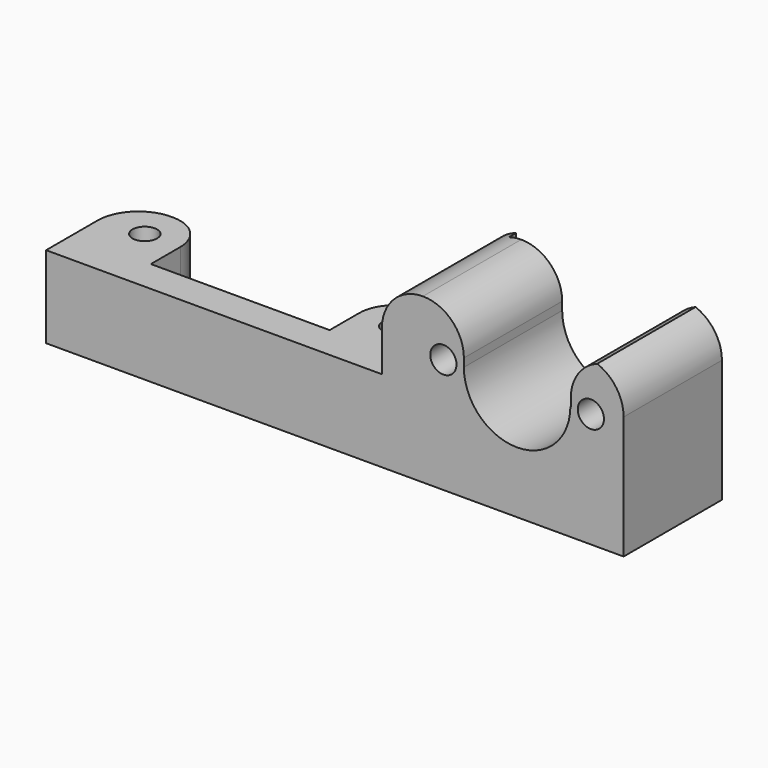
from build123d import *

# Parameters (mm, degrees)
F0_R        = 1.5
F1_DEPTH    = 10
F2_DEPTH    = 20
F4_R        = 1.6
F5_DEPTH    = 15
F6_T1_DEPTH = 40
F6_T3_DEPTH = 41.1
F6_T5_DEPTH = 35.7954738485


# Not quite as in the source:
# - a fillet or chamfer that OpenCascade refuses, or shapes differently, is made with other operations: its cross-section is extruded or revolved along the edge and cut away or added


with BuildPart() as f1:
    # F0 (on Top) → F1 (new body)
    with BuildSketch(Plane.XY):
        with BuildLine():
            Line((-15.25, 4.3355262056), (-20.5, 4.5))
            Line((-20.5, 4.5), (-20.5, -4.5))
            Line((-20.5, -4.5), (-10.9144737944, -4.5))
            Line((-10.9144737944, -4.5), (-10.9144737944, 0))
            ThreePointArc((-10.9144737944, 0), (-12.18432002, 3.06567998), (-15.25, 4.3355262056))
        make_face()
        with Locations((-15.25, 0)):
            Circle(F0_R, mode=Mode.SUBTRACT)
        Polygon((20.5, -8.5), (20.5, -4.5), (10.9144737944, -4.5), (-10.9144737944, -4.5), (-20.5, -4.5), (-20.5, -8.5), align=None)
        with BuildLine():
            Line((20.5, -4.5), (20.5, 4.5))
            Line((20.5, 4.5), (15.25, 4.3355262056))
            ThreePointArc((15.25, 4.3355262056), (12.18432002, 3.06567998), (10.9144737944, 0))
            Line((10.9144737944, 0), (10.9144737944, -4.5))
            Line((10.9144737944, -4.5), (20.5, -4.5))
        make_face()
        with Locations((15.25, 0)):
            Circle(F0_R, mode=Mode.SUBTRACT)
    extrude(amount=F1_DEPTH)


with BuildPart() as f2:
    # F0 (on Top) → F2 (new body)
    with BuildSketch(Plane.XY):
        Polygon((20.5, 7.6), (20.5, 4.5), (20.5, -4.5), (20.5, -8.5), (24, -8.5), (24, 0), (24, 7.6), align=None)
    extrude(amount=F2_DEPTH)


with BuildPart() as f1_1:
    add(f1.part)

    # F3: union F2
    add(f2.part)

    # F4 (on face) → F5 (join)
    with BuildSketch(Plane.XZ.offset(8.5)):
        with BuildLine():
            Line((24, 14), (24, 0))
            Line((24, 0), (50, 0))
            Line((50, 0), (50, 14))
            Line((50, 14), (50, 20))
            Line((50, 20), (43.5623936355, 20))
            Line((43.5623936355, 20), (43.5623936355, 14))
            Line((43.5623936355, 14), (43.5, 14))
            ThreePointArc((43.5, 14), (37, 7.5), (30.5, 14))
            Line((30.5, 14), (30.5, 20))
            Line((30.5, 20), (24, 20))
            Line((24, 20), (24, 14))
        make_face()
        with Locations((28, 14)):
            Circle(F4_R, mode=Mode.SUBTRACT)
        with Locations((46, 14)):
            Circle(F4_R, mode=Mode.SUBTRACT)
    extrude(amount=-F5_DEPTH)

    # F6: fillet of radius 5 on 5 edges, made by hand

    # F6_s2 → F6_t1 (cut)
    with BuildSketch(Plane.XZ.offset(-19)):
        with BuildLine():
            ThreePointArc((43.5623936355, 15), (45.0268597296, 18.5355339059), (48.5623936355, 20))
            Line((48.5623936355, 20), (43.5623936355, 20))
            Line((43.5623936355, 20), (43.5623936355, 15))
        make_face()
        with BuildLine():
            ThreePointArc((45, 20), (48.5355339059, 18.5355339059), (50, 15))
            Line((50, 15), (50, 20))
            Line((50, 20), (45, 20))
        make_face()
        with BuildLine():
            ThreePointArc((30.5, 15), (29.0355339059, 18.5355339059), (25.5, 20))
            Line((25.5, 20), (30.5, 20))
            Line((30.5, 20), (30.5, 15))
        make_face()
    extrude(amount=F6_T1_DEPTH, mode=Mode.SUBTRACT)

    # F6_s4 → F6_t3 (cut)
    with BuildSketch(Plane.XZ.offset(-20.1)):
        with BuildLine():
            ThreePointArc((20.5, 15), (21.9644660941, 18.5355339059), (25.5, 20))
            Line((25.5, 20), (20.5, 20))
            Line((20.5, 20), (20.5, 15))
        make_face()
    extrude(amount=F6_T3_DEPTH, mode=Mode.SUBTRACT)

    # F6_s6 → F6_t5 (cut)
    with BuildSketch(Plane.XY.offset(-12.8977369243)):
        with BuildLine():
            ThreePointArc((-20.5, -0.6590947697), (-18.9797396108, 2.9313665155), (-15.3434351037, 4.3384533725))
            Line((-15.3434351037, 4.3384533725), (-20.5, 4.5))
            Line((-20.5, 4.5), (-20.5, -0.6590947697))
        make_face()
    extrude(amount=F6_T5_DEPTH, mode=Mode.SUBTRACT)


solid = f1_1.part
